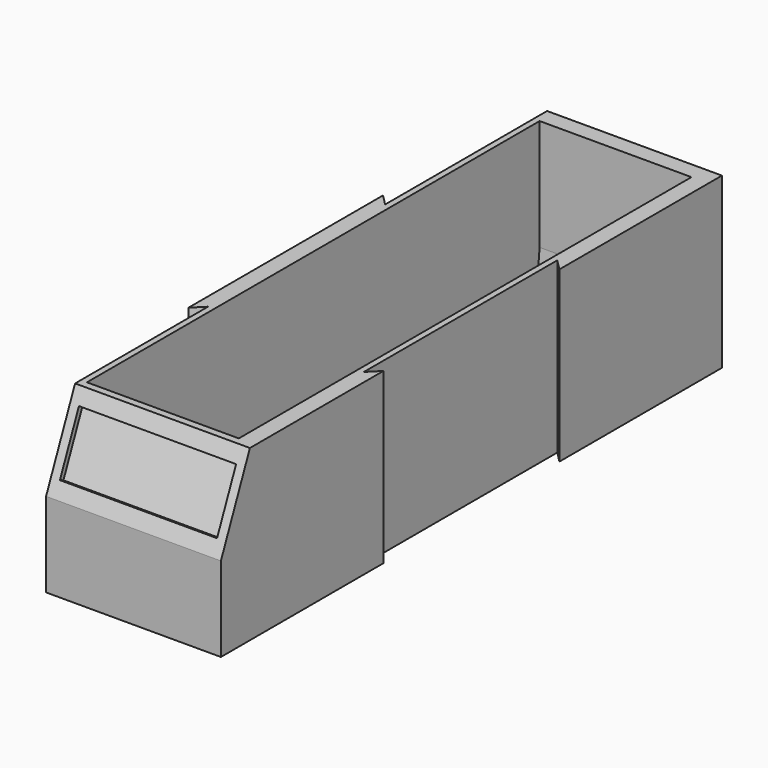
from build123d import *

# Parameters (mm, degrees)
F0_W     = 38.4
F0_H     = 129.5
F0_W_2   = 31.4
F0_H_2   = 111
F1_DEPTH = 2
F2_DEPTH = 35
F3_SIZE2 = 17.5
F3_SIZE  = 7.5
F4_SIZE2 = 32.99999
F4_SIZE  = 5.99999
F6_DEPTH = 35.001
F7_W     = 32.5
F7_H     = 12.5
F8_DEPTH = 1
F9_SIZE2 = 10
F9_SIZE  = 1


# Not quite as in the source:
# - a fillet or chamfer is up to 0.001 mm smaller than in the source, because OpenCascade refuses the exact size


with BuildPart() as f1:
    # F0 (on Top) → F1 (new body)
    with BuildSketch(Plane.XY):
        with Locations((0, -5.75)):
            Rectangle(F0_W, F0_H)
        Rectangle(F0_W_2, F0_H_2, mode=Mode.SUBTRACT)
        Rectangle(F0_W_2, F0_H_2)
    extrude(amount=F1_DEPTH)

    # F0 (on Top) → F2 (join)
    with BuildSketch(Plane.XY):
        with Locations((0, -5.75)):
            Rectangle(F0_W, F0_H)
        Rectangle(F0_W_2, F0_H_2, mode=Mode.SUBTRACT)
    extrude(amount=F2_DEPTH)

    # F3
    f3_edges = [f1.edges().sort_by_distance(p)[0] for p in [
        (0, -70.5, 35),
    ]]
    f3_side = f1.faces().sort_by_distance((0, -69.149266, 35))[0]
    chamfer(f3_edges, length=F3_SIZE, length2=F3_SIZE2, reference=f3_side)

    # F4 (size 6 and 33 in the source; OpenCascade refuses exactly that, so slightly less here)
    f4_edges = [f1.edges().sort_by_distance(p)[0] for p in [
        (0, -55.5, 35),
    ]]
    f4_side = f1.faces().sort_by_distance((17.920994, -2, 35))[0]
    chamfer(f4_edges, length=F4_SIZE, length2=F4_SIZE2, reference=f4_side)

    # F5 (on face) → F6 (cut, through all)
    with BuildSketch(Plane.XY.offset(35)):
        Polygon((19.2, -28.5), (19.2, 17), (16.95, 19.25), (16.95, -30.75), align=None)
        Polygon((-19.2, 19.3914213562), (-16.95, 17.1414213562), (-16.95, 59), (-19.2, 59), align=None)
        Polygon((-16.95, -70.5), (-16.95, -28.6414213562), (-19.2, -30.8914213562), (-19.2, -70.5), align=None)
    extrude(amount=-F6_DEPTH, mode=Mode.SUBTRACT)

    # F7 (on face) → F8 (cut)
    with BuildSketch(Plane(origin=(0, -65.8965517241, 28.2413793103), x_dir=(1, 0, 0), z_dir=(0, -0.91914503, 0.3939192986))):
        with Locations((1.125, -2.1665561422)):
            Rectangle(F7_W, F7_H)
    extrude(amount=-F8_DEPTH, mode=Mode.SUBTRACT)

    # F9
    f9_edges = [f1.edges().sort_by_distance(p)[0] for p in [
        (0, 55.5, 2),
    ]]
    f9_side = f1.faces().sort_by_distance((0, 0, 2))[0]
    chamfer(f9_edges, length=F9_SIZE, length2=F9_SIZE2, reference=f9_side)


solid = f1.part
